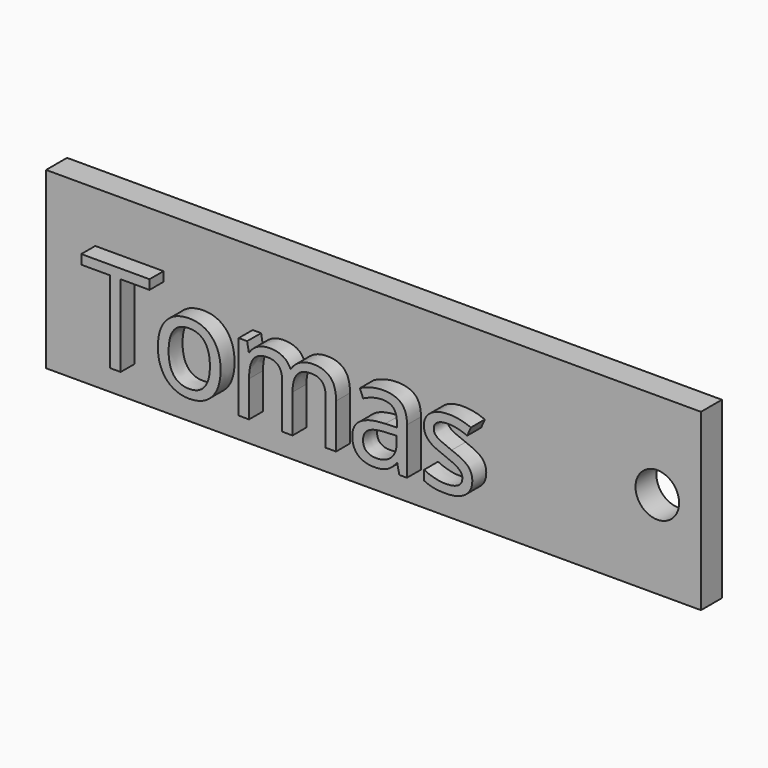
from build123d import *

# Parameters (mm, degrees)
F0_W         = 75
F0_H         = 20
F0_R         = 2.5
F1_DEPTH     = 3
F2_TEXT_SIZE = 14.6059785038
F3_DEPTH     = 2


# Not quite as in the source:
# - Text() gives the source's letters only with a copy of the font that has no kerning and outlines rounded to 1/6400 em; it was checked with that copy


with BuildPart() as f1:
    # F0 (on Front) → F1 (new body)
    with BuildSketch(Plane.XZ):
        with Locations((37.5, -10)):
            Rectangle(F0_W, F0_H)
        with Locations((70, -10)):
            Circle(F0_R, mode=Mode.SUBTRACT)
    extrude(amount=F1_DEPTH)

    # F2 (on face) → F3 (join)
    with BuildSketch(Plane.XZ.offset(3)):
        with Locations((5.5027166381, -16.2635874003)):
            Text('Tomas', F2_TEXT_SIZE, font='Open Sans', text_align=(TextAlign.LEFT, TextAlign.BOTTOM))
    extrude(amount=F3_DEPTH)


solid = f1.part
